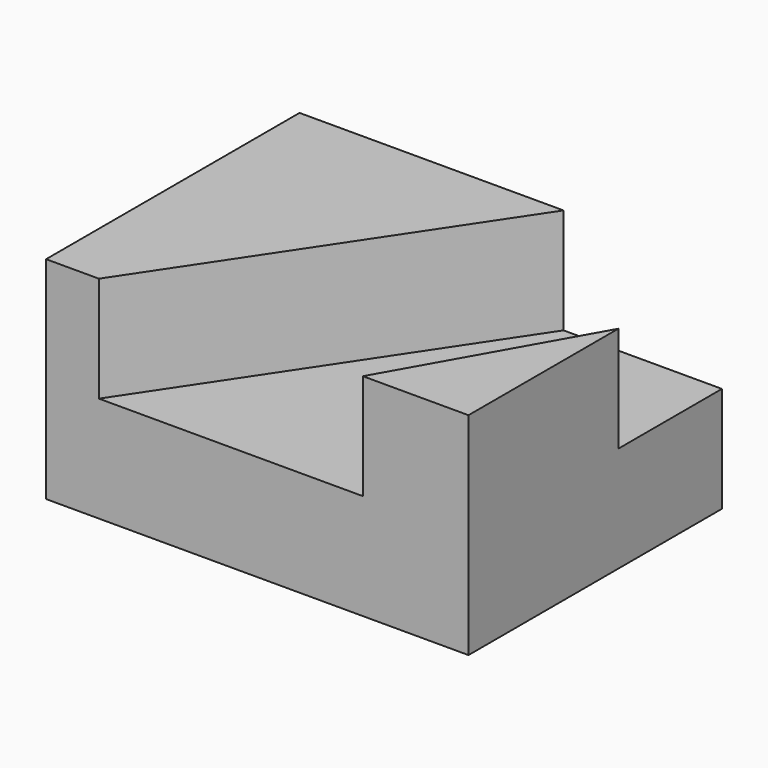
from build123d import *

# Parameters (mm, degrees)
F0_W     = 101.6
F0_H     = 76.2
F1_DEPTH = 25.4
F5_DEPTH = 25.4
F8_DEPTH = 25.4


# Not quite as in the source:
# - a feature of the source that left no trace in its solid (it failed there, or was rolled back) is left out


with BuildPart() as f1:
    # F0 (on Top) → F1 (new body)
    with BuildSketch(Plane.XY):
        with Locations((-10.3016215888, -18.0514037281)):
            Rectangle(F0_W, F0_H)
    extrude(amount=F1_DEPTH)

    # F4 (on face) → F5 (join)
    with BuildSketch(Plane.XY.offset(25.4)):
        Polygon((15.0983784112, -56.1514037281), (40.4983784112, -56.1514037281), (40.4983784112, -11.0943727195), align=None)
    extrude(amount=F5_DEPTH)

    # F7 (on face) → F8 (join)
    with BuildSketch(Plane.XY.offset(25.4)):
        Polygon((-61.1016215888, -56.1514037281), (-48.4016215888, -56.1514037281), (2.3983784112, 20.0485962719), (-61.1016215888, 20.0485962719), align=None)
    extrude(amount=F8_DEPTH)


solid = f1.part
